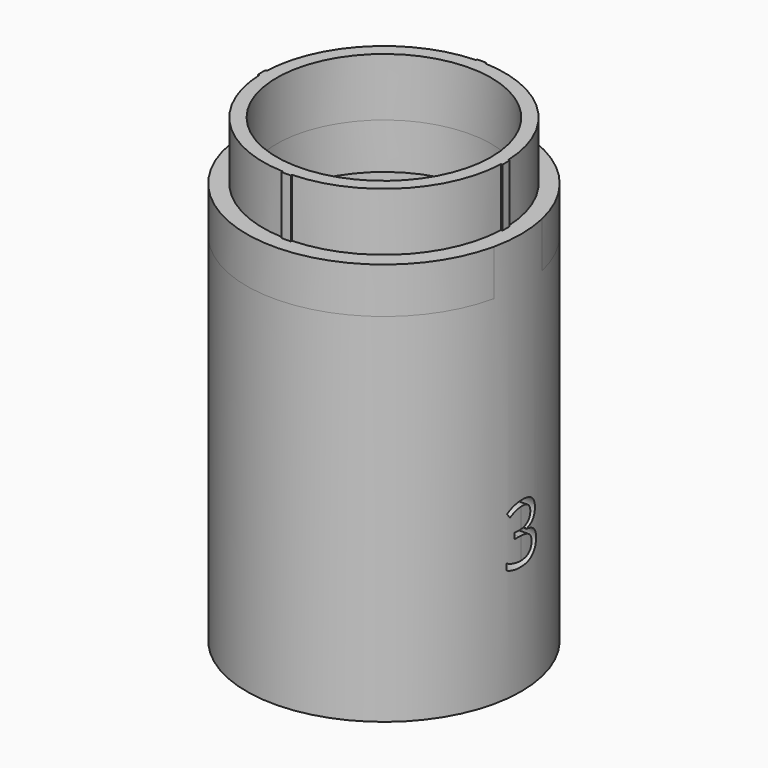
from build123d import *

# Parameters (mm, degrees)
F0_R         = 11.725
F1_DEPTH     = 6.35
F2_R         = 15
F2_R_2       = 13.35
F3_DEPTH     = 44
F4_R         = 15
F4_R_2       = 11.725
F5_DEPTH     = 5
F6_TEXT_SIZE = 8.7370552743
F7_DEPTH     = 25


# Not quite as in the source:
# - Text() gives the source's letters only with a copy of the font that has no kerning and outlines rounded to 1/6400 em; it was checked with that copy


with BuildPart() as f1:
    # F0 (on Top) → F1 (new body)
    with BuildSketch(Plane.XY):
        with BuildLine():
            ThreePointArc((13.1905269038, -0.5), (13.1976315135, -0.2500448657), (13.2, 0))
            ThreePointArc((13.2, 0), (13.1976315135, 0.2500448657), (13.1905269038, 0.5))
            ThreePointArc((13.1905269038, 0.5), (9.3338095117, 9.3338095117), (0.5, 13.1905269038))
            ThreePointArc((0.5, 13.1905269038), (0, 13.2), (-0.5, 13.1905269038))
            ThreePointArc((-0.5, 13.1905269038), (-9.3338095117, 9.3338095117), (-13.1905269038, 0.5))
            ThreePointArc((-13.1905269038, 0.5), (-13.2, 0), (-13.1905269038, -0.5))
            ThreePointArc((-13.1905269038, -0.5), (-9.3338095117, -9.3338095117), (-0.5, -13.1905269038))
            ThreePointArc((-0.5, -13.1905269038), (0, -13.2), (0.5, -13.1905269038))
            ThreePointArc((0.5, -13.1905269038), (9.3338095117, -9.3338095117), (13.1905269038, -0.5))
        make_face()
        Circle(F0_R, mode=Mode.SUBTRACT)
        with BuildLine():
            ThreePointArc((13.1905269038, 0.5), (13.1976315135, 0.2500448657), (13.2, 0))
            ThreePointArc((13.2, 0), (13.1976315135, -0.2500448657), (13.1905269038, -0.5))
            Line((13.1905269038, -0.5), (13.3406334182, -0.5))
            ThreePointArc((13.3406334182, -0.5), (13.35, 0), (13.3406334182, 0.5))
            Line((13.3406334182, 0.5), (13.1905269038, 0.5))
        make_face()
        with BuildLine():
            ThreePointArc((-0.5, 13.1905269038), (0, 13.2), (0.5, 13.1905269038))
            Line((0.5, 13.1905269038), (0.5, 13.3406334182))
            ThreePointArc((0.5, 13.3406334182), (0, 13.35), (-0.5, 13.3406334182))
            Line((-0.5, 13.3406334182), (-0.5, 13.1905269038))
        make_face()
        with BuildLine():
            Line((0.5, -13.3406334182), (0.5, -13.1905269038))
            ThreePointArc((0.5, -13.1905269038), (0, -13.2), (-0.5, -13.1905269038))
            Line((-0.5, -13.1905269038), (-0.5, -13.3406334182))
            ThreePointArc((-0.5, -13.3406334182), (0, -13.35), (0.5, -13.3406334182))
        make_face()
        with BuildLine():
            ThreePointArc((-13.1905269038, -0.5), (-13.2, 0), (-13.1905269038, 0.5))
            Line((-13.1905269038, 0.5), (-13.3406334182, 0.5))
            ThreePointArc((-13.3406334182, 0.5), (-13.35, 0), (-13.3406334182, -0.5))
            Line((-13.3406334182, -0.5), (-13.1905269038, -0.5))
        make_face()
    extrude(amount=F1_DEPTH)

    # F2 (on Top) → F3 (join)
    with BuildSketch(Plane.XY):
        Circle(F2_R)
        Circle(F2_R_2, mode=Mode.SUBTRACT)
    extrude(amount=-F3_DEPTH)

    # F6 (on Right) → F7 (cut)
    with BuildSketch(Plane.YZ):
        with Locations((-2.2416007438, -31.9193787873)):
            Text('3', F6_TEXT_SIZE, font='Open Sans', text_align=(TextAlign.LEFT, TextAlign.BOTTOM))
    extrude(amount=F7_DEPTH, mode=Mode.SUBTRACT)


with BuildPart() as f5:
    # F4 (on Top) → F5 (new body)
    with BuildSketch(Plane.XY):
        Circle(F4_R)
        Circle(F4_R_2, mode=Mode.SUBTRACT)
    extrude(amount=-F5_DEPTH)


solid = Compound([f1.part, f5.part])
